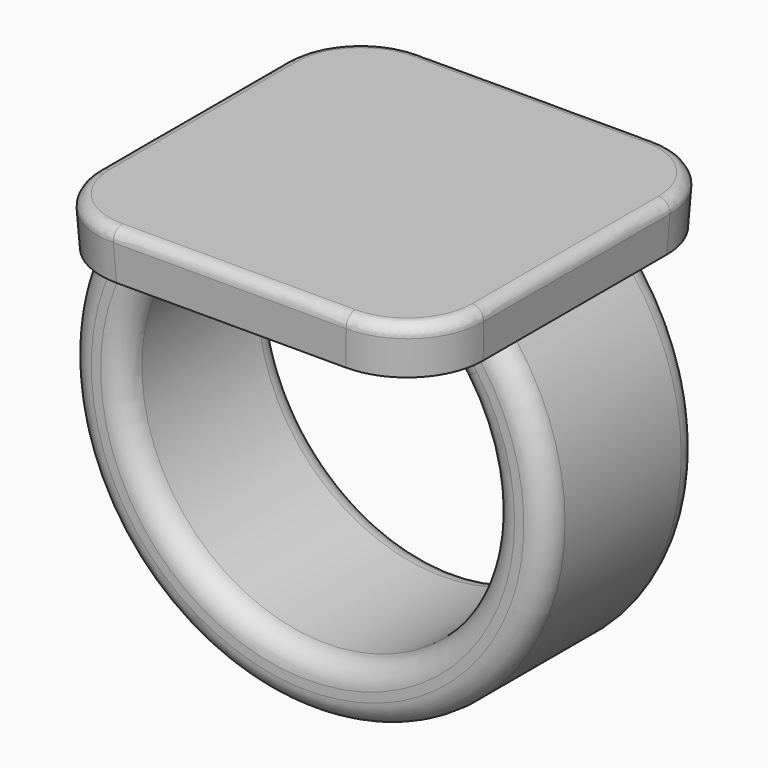
from build123d import *

# Parameters (mm, degrees)
F0_W          = 25.4
F0_H          = 25.4
F1_DEPTH      = 3.175
F1_TAPER      = -3
F3_W          = 5.08
F3_H          = 12.7
F6_DEPTH      = 6.35
F6_DEPTH_BACK = 6.35
F7_R          = 5.08
F8_R          = 1.524
F9_R          = 0.762


with BuildPart() as f1:
    # F0 (on Top) → F1 (new body)
    with BuildSketch(Plane.XY):
        Rectangle(F0_W, F0_H)
    extrude(amount=F1_DEPTH, taper=F1_TAPER)

    # F4: sweep along a path in F2
    with BuildLine(Plane.XZ) as f4_path:
        ThreePointArc((-10.16, 0), (0, -23.5582897328), (10.16, 0))
    # F3 (on face) → F4 (sweep)
    with BuildSketch(Plane(origin=(0, 0, 0), x_dir=(1, 0, 0), z_dir=(0, 0, -1))):
        with Locations((-10.16, 0)):
            Rectangle(F3_W, F3_H)
    sweep(path=f4_path.line)

    # F5 (on Front) → F6 (join, two sides)
    with BuildSketch(Plane.XZ) as f6_sk:
        with BuildLine():
            ThreePointArc((7.62, 0), (8.9072265211, -1.1822790439), (10.0130578512, -2.535746045))
            Line((10.0130578512, -2.535746045), (10.16, 0))
            Line((10.16, 0), (7.62, 0))
        make_face()
    extrude(amount=F6_DEPTH)
    extrude(f6_sk.sketch, amount=-F6_DEPTH_BACK)

    # F7
    f7_edges = [f1.edges().sort_by_distance(p)[0] for p in [
        (12.783197, 12.783197, 1.5875),
        (12.783197, -12.783197, 1.5875),
        (-12.783197, -12.783197, 1.5875),
        (-12.783197, 12.783197, 1.5875),
    ]]
    fillet(f7_edges, radius=F7_R)

    # F8
    f8_edges = [f1.edges().sort_by_distance(p)[0] for p in [
        (-1.743325, 6.35, -21.711017),
        (8.907227, 6.35, -1.182279),
        (-1.743325, -6.35, -21.711017),
        (0, 6.35, -25.501344),
        (0, -6.35, -25.501344),
        (8.907227, -6.35, -1.182279),
    ]]
    fillet(f8_edges, radius=F8_R)

    # F9
    f9_edges = [f1.edges().sort_by_distance(p)[0] for p in [
        (-12.866395, 0, 3.175),
        (-11.381378, 11.381378, 3.175),
        (-11.381378, -11.381378, 3.175),
        (0, 12.866395, 3.175),
        (0, -12.866395, 3.175),
        (11.381378, 11.381378, 3.175),
        (11.381378, -11.381378, 3.175),
        (12.866395, 0, 3.175),
    ]]
    fillet(f9_edges, radius=F9_R)


solid = f1.part
